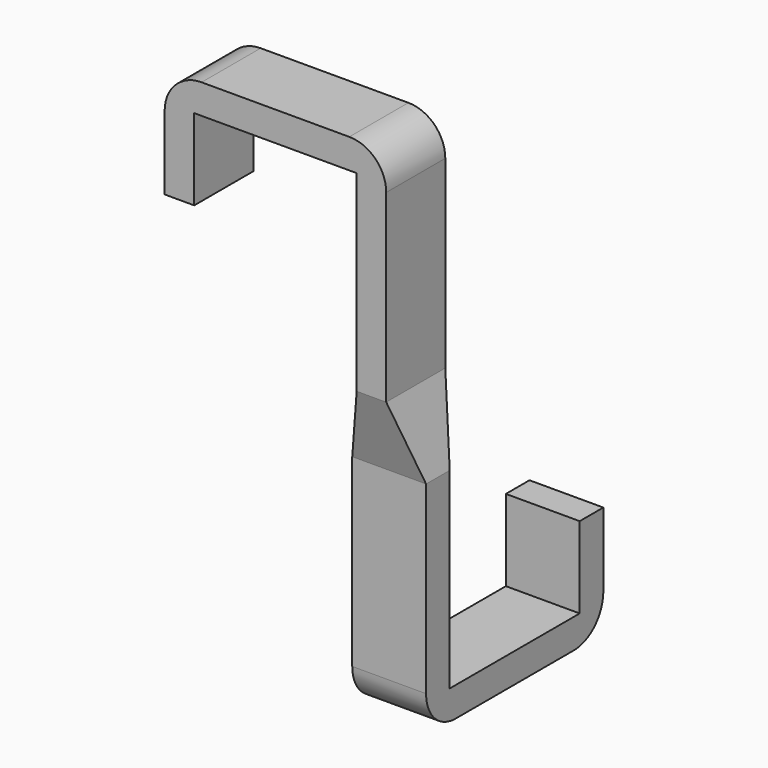
from build123d import *

# Parameters (mm, degrees)
F1_DEPTH  = 10
F2_ANGLE  = 180
F3_ANGLE  = 90
F2_FACE_W = 10
F2_FACE_H = 4
F1_FACE_W = 4
F1_FACE_H = 10


with BuildPart() as f1:
    # F0 (on Front) → F1 (new body)
    with BuildSketch(Plane.XZ):
        with BuildLine():
            Line((-33.0547787249, 16.2792187184), (-53.0547787249, 16.2792187184))
            ThreePointArc((-53.0547787249, 16.2792187184), (-56.5903126308, 14.8147526243), (-58.0547787249, 11.2792187184))
            Line((-58.0547787249, 11.2792187184), (-58.0547787249, 1.2792187184))
            Line((-58.0547787249, 1.2792187184), (-54.0547787249, 1.2792187184))
            Line((-54.0547787249, 1.2792187184), (-54.0547787249, 12.2792187184))
            Line((-54.0547787249, 12.2792187184), (-32.0547787249, 12.2792187184))
            Line((-32.0547787249, 12.2792187184), (-32.0547787249, -13.7207812816))
            Line((-32.0547787249, -13.7207812816), (-28.0547787249, -13.7207812816))
            Line((-28.0547787249, -13.7207812816), (-28.0547787249, 11.2792187184))
            ThreePointArc((-28.0547787249, 11.2792187184), (-29.519244819, 14.8147526243), (-33.0547787249, 16.2792187184))
        make_face()
    extrude(amount=F1_DEPTH)


with BuildPart() as f2_1:
    # F2: copy of F1
    add(f1.part.rotate(Axis((-28.0547787249, -5, -13.7207812816), (0, 1, 0)), F2_ANGLE))


with BuildPart() as f2_1_1:
    # F3: moved
    add(f2_1.part.rotate(Axis((-28.0547787249, 0, -26.2207812816), (0, 0, 1)), F3_ANGLE))


with BuildPart() as f2_1_2:
    # F4: moved
    add(f2_1_1.part.moved(Location((-7, -7, -10))))

    # F2_face (on face) → F5 section 0
    with BuildSketch(Plane(origin=(-30.0547787249, -5, -23.7207812816), x_dir=(1, 0, 0), z_dir=(0, 0, 1))):
        Rectangle(F2_FACE_W, F2_FACE_H)
    # F1_face (on face) → F5 section 1
    with BuildSketch(Plane(origin=(-30.0547787249, -5, -13.7207812816), x_dir=(1, 0, 0), z_dir=(0, 0, -1))):
        Rectangle(F1_FACE_W, F1_FACE_H)
    loft()


solid = Compound([f1.part, f2_1_2.part])
